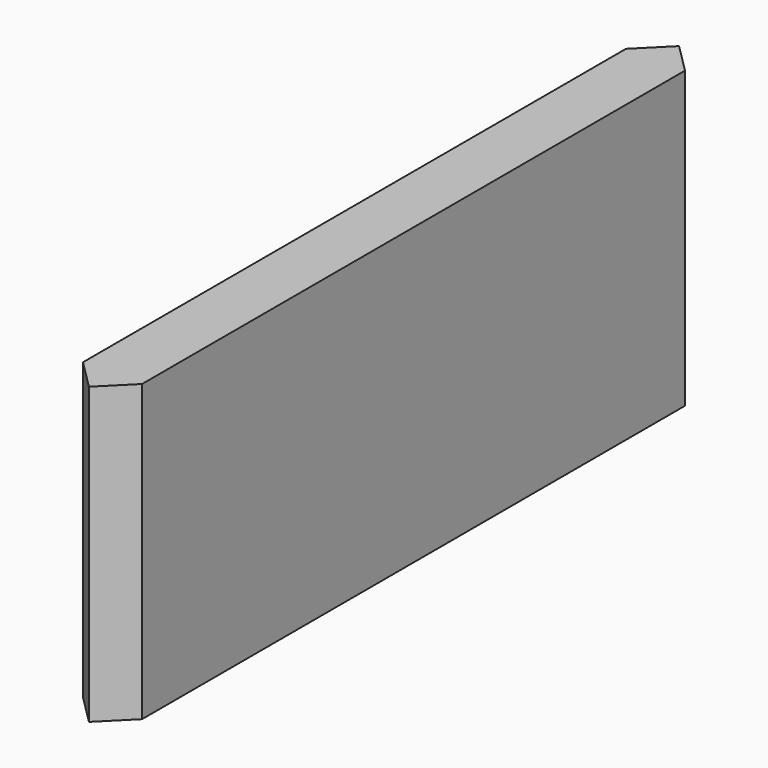
from build123d import *

# Parameters (mm, degrees)
F0_W     = 75
F0_H     = 30
F1_DEPTH = 3
F2_SIZE  = 2.99999


# Not quite as in the source:
# - a fillet or chamfer is up to 0.001 mm smaller than in the source, because OpenCascade refuses the exact size


with BuildPart() as f1:
    # F0 (on Right) → F1 (new body, symmetric)
    with BuildSketch(Plane.YZ):
        with Locations((0, 15)):
            Rectangle(F0_W, F0_H)
    extrude(amount=F1_DEPTH, both=True)

    # F2 (size 3 in the source; OpenCascade refuses exactly that, so slightly less here)
    f2_edges = [f1.edges().sort_by_distance(p)[0] for p in [
        (3, -37.5, 15),
        (-3, -37.5, 15),
        (-3, 37.5, 15),
        (3, 37.5, 15),
    ]]
    chamfer(f2_edges, length=F2_SIZE)


solid = f1.part
